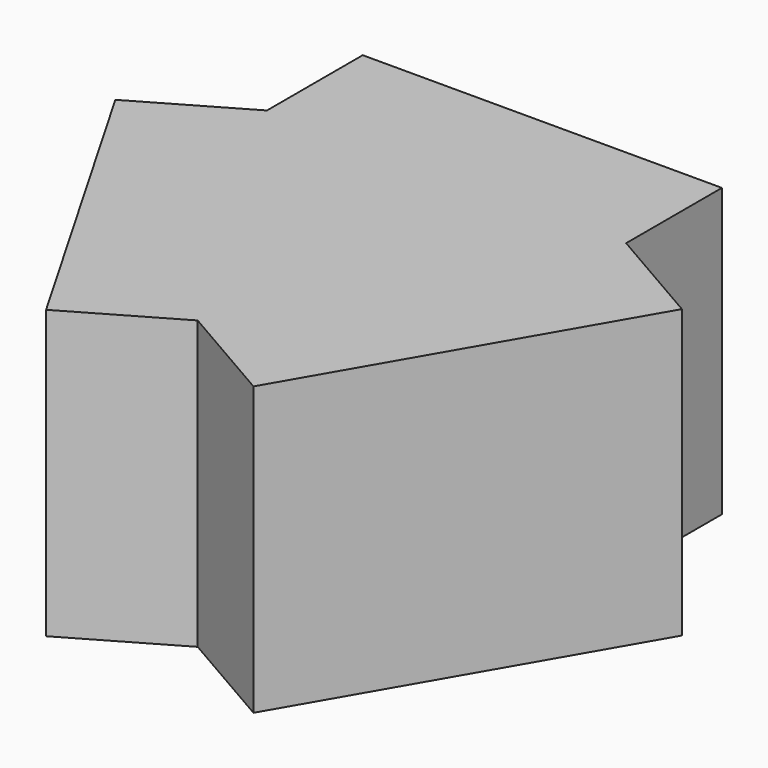
from build123d import *

# Parameters (mm, degrees)
F1_DEPTH = 18
F2_DEPTH = 15
F3_DEPTH = 15
F4_DEPTH = 15


# Not quite as in the source:
# - the program builds the solid bodies; features that only make, move or delete a surface that nothing else refers to are left out


with BuildPart() as f1:
    # F0 (on Top) → F1 (new body, symmetric)
    with BuildSketch(Plane.XY):
        Polygon((22.5, 12.9903810568), (-22.5, 12.9903810568), (0, -25.9807621135), align=None)
    extrude(amount=F1_DEPTH, both=True)

    # F2 (add): a face of the model
    f2_faces = [f1.faces().sort_by_distance(p)[0] for p in [
        (11.25, -6.4951905284, 0),
    ]]
    extrude(f2_faces, amount=F2_DEPTH)

    # F3 (add): a face of the model
    f3_faces = [f1.faces().sort_by_distance(p)[0] for p in [
        (0, 12.9903810568, 0),
    ]]
    extrude(f3_faces, amount=F3_DEPTH)

    # F4 (add): a face of the model
    f4_faces = [f1.faces().sort_by_distance(p)[0] for p in [
        (-11.25, -6.4951905284, 0),
    ]]
    extrude(f4_faces, amount=F4_DEPTH)


solid = f1.part
